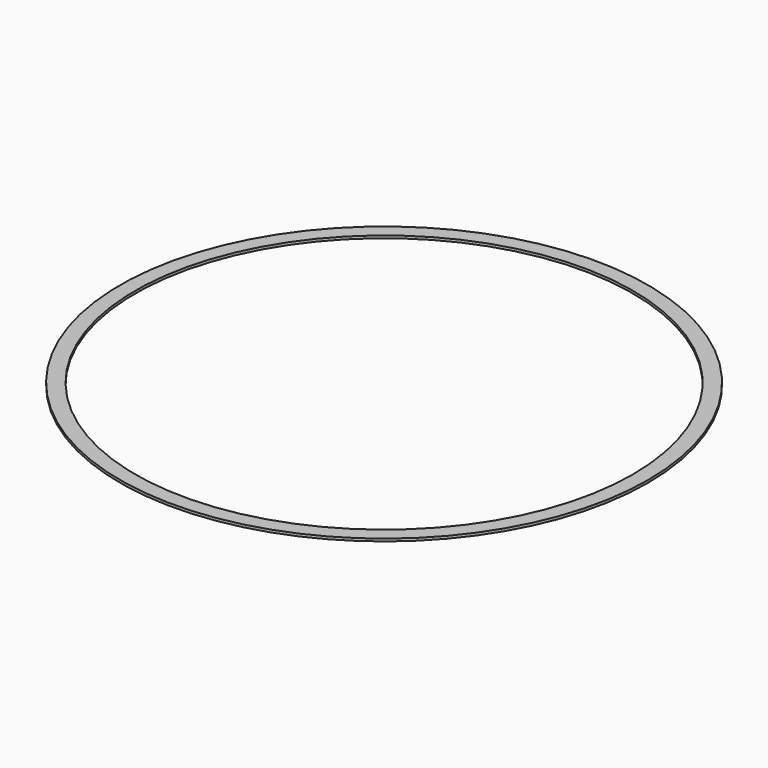
from build123d import *

# Parameters (mm, degrees)
F0_R     = 442.04636
F0_R_2   = 416.64636
F1_DEPTH = 4.2333333333


# Not quite as in the source:
# - a length typed as a fraction of an inch, garbled in the dataset ("3 / 203.2 mm" for 3/8 in), is restored


with BuildPart() as f1:
    # F0 (on Top) → F1 (new body)
    with BuildSketch(Plane.XY):
        Circle(F0_R)
        Circle(F0_R_2, mode=Mode.SUBTRACT)
    extrude(amount=F1_DEPTH)


solid = f1.part
